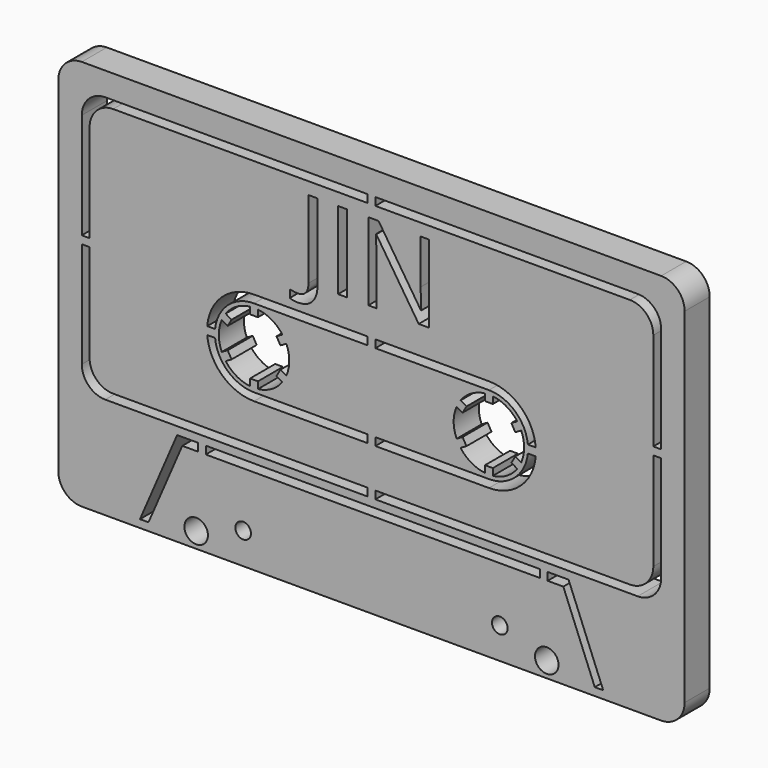
from build123d import *

# Parameters (mm, degrees)
F0_R         = 1.905
F0_R_2       = 1.27
F0_W         = 54.1864509355
F0_H         = 1.27
F1_DEPTH     = 5.08
F2_TEXT_SIZE = 17.6388888889
F3_DEPTH     = 25.4


# Not quite as in the source:
# - Text() gives the source's letters only with a copy of the font that has no kerning and outlines rounded to 1/6400 em; it was checked with that copy


with BuildPart() as f1:
    # F0 (on Front) → F1 (new body)
    with BuildSketch(Plane.XZ):
        with BuildLine():
            ThreePointArc((50.8, 27.94), (49.6840768363, 30.6340768363), (46.99, 31.75))
            Line((46.99, 31.75), (-46.99, 31.75))
            ThreePointArc((-46.99, 31.75), (-49.6840768363, 30.6340768363), (-50.8, 27.94))
            Line((-50.8, 27.94), (-50.8, -27.94))
            ThreePointArc((-50.8, -27.94), (-49.6840768363, -30.6340768363), (-46.99, -31.75))
            Line((-46.99, -31.75), (46.99, -31.75))
            ThreePointArc((46.99, -31.75), (49.6840768363, -30.6340768363), (50.8, -27.94))
            Line((50.8, -27.94), (50.8, 27.94))
        make_face()
        with Locations((-28.4354059759, -29.21)):
            Circle(F0_R, mode=Mode.SUBTRACT)
        Polygon((-36.1690502777, -30.48), (-37.5521693637, -30.48), (-31.5260323644, -16.51), (-28.1507439147, -16.51), (-28.1507439147, -17.78), (-30.6907439147, -17.78), align=None, mode=Mode.SUBTRACT)
        with Locations((-20.8154059759, -26.67)):
            Circle(F0_R_2, mode=Mode.SUBTRACT)
        with BuildLine():
            Line((-0.635, -15.24), (-43.18, -15.24))
            ThreePointArc((-43.18, -15.24), (-45.8740768363, -14.1240768363), (-46.99, -11.43))
            Line((-46.99, -11.43), (-46.99, 5.715))
            Line((-46.99, 5.715), (-45.72, 5.715))
            Line((-45.72, 5.715), (-45.72, -10.16))
            ThreePointArc((-45.72, -10.16), (-44.6040768363, -12.8540768363), (-41.91, -13.97))
            Line((-41.91, -13.97), (-0.635, -13.97))
            Line((-0.635, -13.97), (-0.635, -15.24))
        make_face(mode=Mode.SUBTRACT)
        with BuildLine():
            ThreePointArc((-25.3681702256, -0.635), (-23.3097094971, -4.7092860393), (-19.05, -6.35))
            Line((-19.05, -6.35), (-0.635, -6.35))
            Line((-0.635, -6.35), (-0.635, -7.62))
            Line((-0.635, -7.62), (-19.05, -7.62))
            ThreePointArc((-19.05, -7.62), (-24.2087643869, -5.6081681501), (-26.6434955719, -0.635))
            Line((-26.6434955719, -0.635), (-25.3681702256, -0.635))
        make_face(mode=Mode.SUBTRACT)
        with Locations((20.8154059759, -26.67)):
            Circle(F0_R_2, mode=Mode.SUBTRACT)
        with Locations((0.2124815531, -17.145)):
            Rectangle(F0_W, F0_H, mode=Mode.SUBTRACT)
        with Locations((28.4354059759, -29.21)):
            Circle(F0_R, mode=Mode.SUBTRACT)
        Polygon((28.5757070209, -16.51), (31.9739676356, -16.51), (37.589497303, -30.48), (36.2207339912, -30.48), (31.1157070209, -17.78), (28.5757070209, -17.78), align=None, mode=Mode.SUBTRACT)
        with BuildLine():
            Line((0.635, -7.62), (0.635, -6.35))
            Line((0.635, -6.35), (19.05, -6.35))
            ThreePointArc((19.05, -6.35), (23.3097094971, -4.7092860393), (25.3681702256, -0.635))
            Line((25.3681702256, -0.635), (26.6434955719, -0.635))
            ThreePointArc((26.6434955719, -0.635), (24.2087643869, -5.6081681501), (19.05, -7.62))
            Line((19.05, -7.62), (0.635, -7.62))
        make_face(mode=Mode.SUBTRACT)
        with BuildLine():
            ThreePointArc((46.99, -11.43), (45.8740768363, -14.1240768363), (43.18, -15.24))
            Line((43.18, -15.24), (0.635, -15.24))
            Line((0.635, -15.24), (0.635, -13.97))
            Line((0.635, -13.97), (41.91, -13.97))
            ThreePointArc((41.91, -13.97), (44.6040768363, -12.8540768363), (45.72, -10.16))
            Line((45.72, -10.16), (45.72, 5.715))
            Line((45.72, 5.715), (46.99, 5.715))
            Line((46.99, 5.715), (46.99, -11.43))
        make_face(mode=Mode.SUBTRACT)
        with BuildLine():
            ThreePointArc((-23.6511888497, 3.3897324628), (-21.9075, 4.9493351826), (-19.685, 5.6796126628))
            Line((-19.685, 5.6796126628), (-19.685, 4.572))
            Line((-19.685, 4.572), (-18.415, 4.572))
            Line((-18.415, 4.572), (-18.415, 5.6796126628))
            ThreePointArc((-18.415, 5.6796126628), (-16.1925, 4.9493351826), (-14.4488111503, 3.3897324628))
            Line((-14.4488111503, 3.3897324628), (-15.4080318539, 2.8359261314))
            Line((-15.4080318539, 2.8359261314), (-14.7730318539, 1.7360738686))
            Line((-14.7730318539, 1.7360738686), (-13.8138111503, 2.2898802))
            ThreePointArc((-13.8138111503, 2.2898802), (-13.335, 0), (-13.8138111503, -2.2898802))
            Line((-13.8138111503, -2.2898802), (-14.7730318539, -1.7360738686))
            Line((-14.7730318539, -1.7360738686), (-15.4080318539, -2.8359261314))
            Line((-15.4080318539, -2.8359261314), (-14.4488111503, -3.3897324628))
            ThreePointArc((-14.4488111503, -3.3897324628), (-16.1925, -4.9493351826), (-18.415, -5.6796126628))
            Line((-18.415, -5.6796126628), (-18.415, -4.572))
            Line((-18.415, -4.572), (-19.685, -4.572))
            Line((-19.685, -4.572), (-19.685, -5.6796126628))
            ThreePointArc((-19.685, -5.6796126628), (-21.9075, -4.9493351826), (-23.6511888497, -3.3897324628))
            Line((-23.6511888497, -3.3897324628), (-22.6919681461, -2.8359261314))
            Line((-22.6919681461, -2.8359261314), (-23.3269681461, -1.7360738686))
            Line((-23.3269681461, -1.7360738686), (-24.2861888497, -2.2898802))
            ThreePointArc((-24.2861888497, -2.2898802), (-24.765, 0), (-24.2861888497, 2.2898802))
            Line((-24.2861888497, 2.2898802), (-23.3269681461, 1.7360738686))
            Line((-23.3269681461, 1.7360738686), (-22.6919681461, 2.8359261314))
            Line((-22.6919681461, 2.8359261314), (-23.6511888497, 3.3897324628))
        make_face(mode=Mode.SUBTRACT)
        with BuildLine():
            Line((-0.635, 6.35), (-19.05, 6.35))
            ThreePointArc((-19.05, 6.35), (-23.3097094971, 4.7092860393), (-25.3681702256, 0.635))
            Line((-25.3681702256, 0.635), (-26.6434955719, 0.635))
            ThreePointArc((-26.6434955719, 0.635), (-24.2087643869, 5.6081681501), (-19.05, 7.62))
            Line((-19.05, 7.62), (-0.635, 7.62))
            Line((-0.635, 7.62), (-0.635, 6.35))
        make_face(mode=Mode.SUBTRACT)
        with BuildLine():
            ThreePointArc((-46.99, 24.13), (-45.8740768363, 26.8240768363), (-43.18, 27.94))
            Line((-43.18, 27.94), (-0.635, 27.94))
            Line((-0.635, 27.94), (-0.635, 26.67))
            Line((-0.635, 26.67), (-41.91, 26.67))
            ThreePointArc((-41.91, 26.67), (-44.6040768363, 25.5540768363), (-45.72, 22.86))
            Line((-45.72, 22.86), (-45.72, 6.985))
            Line((-45.72, 6.985), (-46.99, 6.985))
            Line((-46.99, 6.985), (-46.99, 24.13))
        make_face(mode=Mode.SUBTRACT)
        with BuildLine():
            ThreePointArc((14.4488111503, 3.3897324628), (16.1925, 4.9493351826), (18.415, 5.6796126628))
            Line((18.415, 5.6796126628), (18.415, 4.572))
            Line((18.415, 4.572), (19.685, 4.572))
            Line((19.685, 4.572), (19.685, 5.6796126628))
            ThreePointArc((19.685, 5.6796126628), (21.9075, 4.9493351826), (23.6511888497, 3.3897324628))
            Line((23.6511888497, 3.3897324628), (22.6919681461, 2.8359261314))
            Line((22.6919681461, 2.8359261314), (23.3269681461, 1.7360738686))
            Line((23.3269681461, 1.7360738686), (24.2861888497, 2.2898802))
            ThreePointArc((24.2861888497, 2.2898802), (24.765, 0), (24.2861888497, -2.2898802))
            Line((24.2861888497, -2.2898802), (23.3269681461, -1.7360738686))
            Line((23.3269681461, -1.7360738686), (22.6919681461, -2.8359261314))
            Line((22.6919681461, -2.8359261314), (23.6511888497, -3.3897324628))
            ThreePointArc((23.6511888497, -3.3897324628), (21.9075, -4.9493351826), (19.685, -5.6796126628))
            Line((19.685, -5.6796126628), (19.685, -4.572))
            Line((19.685, -4.572), (18.415, -4.572))
            Line((18.415, -4.572), (18.415, -5.6796126628))
            ThreePointArc((18.415, -5.6796126628), (16.1925, -4.9493351826), (14.4488111503, -3.3897324628))
            Line((14.4488111503, -3.3897324628), (15.4080318539, -2.8359261314))
            Line((15.4080318539, -2.8359261314), (14.7730318539, -1.7360738686))
            Line((14.7730318539, -1.7360738686), (13.8138111503, -2.2898802))
            ThreePointArc((13.8138111503, -2.2898802), (13.335, 0), (13.8138111503, 2.2898802))
            Line((13.8138111503, 2.2898802), (14.7730318539, 1.7360738686))
            Line((14.7730318539, 1.7360738686), (15.4080318539, 2.8359261314))
            Line((15.4080318539, 2.8359261314), (14.4488111503, 3.3897324628))
        make_face(mode=Mode.SUBTRACT)
        with BuildLine():
            Line((0.635, 6.35), (0.635, 7.62))
            Line((0.635, 7.62), (19.05, 7.62))
            ThreePointArc((19.05, 7.62), (21.2497045256, 7.2955945611), (23.2621134838, 6.35))
            ThreePointArc((23.2621134838, 6.35), (25.6080795622, 3.880205208), (26.6434955719, 0.635))
            Line((26.6434955719, 0.635), (25.3681702256, 0.635))
            ThreePointArc((25.3681702256, 0.635), (23.3097094971, 4.7092860393), (19.05, 6.35))
            Line((19.05, 6.35), (0.635, 6.35))
        make_face(mode=Mode.SUBTRACT)
        with BuildLine():
            ThreePointArc((43.18, 27.94), (45.8740768363, 26.8240768363), (46.99, 24.13))
            Line((46.99, 24.13), (46.99, 6.985))
            Line((46.99, 6.985), (45.72, 6.985))
            Line((45.72, 6.985), (45.72, 22.86))
            ThreePointArc((45.72, 22.86), (44.6040768363, 25.5540768363), (41.91, 26.67))
            Line((41.91, 26.67), (0.635, 26.67))
            Line((0.635, 26.67), (0.635, 27.94))
            Line((0.635, 27.94), (43.18, 27.94))
        make_face(mode=Mode.SUBTRACT)
    extrude(amount=F1_DEPTH)

    # F2 (on face) → F3 (cut)
    with BuildSketch(Plane.XZ.offset(5.08)):
        with Locations((-11.8618, 12.1012137619)):
            Text('JIN', F2_TEXT_SIZE, font='Open Sans', text_align=(TextAlign.LEFT, TextAlign.BOTTOM))
    extrude(amount=-F3_DEPTH, mode=Mode.SUBTRACT)


solid = f1.part
